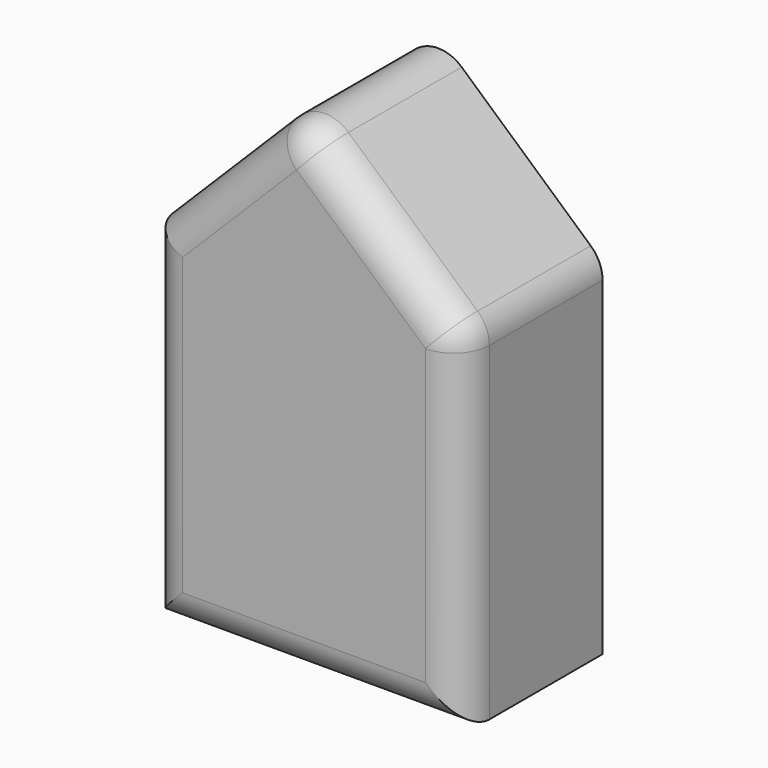
from build123d import *

# Parameters (mm, degrees)
F0_W     = 45.0788065791
F0_H     = 49.5671723038
F1_DEPTH = 25.4
F3_R     = 5.08


# Not quite as in the source:
# - a feature of the source that left no trace in its solid (it failed there, or was rolled back) is left out


with BuildPart() as f1:
    # F0 (on Front) → F1 (new body)
    with BuildSketch(Plane.XZ):
        with Locations((-4.0004998446, -2.9271943495)):
            Rectangle(F0_W, F0_H)
        Polygon((-5.2689509466, 43.1273430586), (-26.5399031341, 21.8563918024), (18.538903445, 21.8563918024), align=None)
    extrude(amount=F1_DEPTH)

    # F3
    f3_edges = [f1.edges().sort_by_distance(p)[0] for p in [
        (-15.904427, -25.4, 32.491867),
        (-26.539903, -25.4, -2.927194),
        (-4.0005, -25.4, -27.710781),
        (18.538903, -25.4, -2.927194),
        (6.634976, -25.4, 32.491867),
        (18.538903, -12.7, 21.856392),
        (-5.268951, -12.7, 43.127343),
    ]]
    fillet(f3_edges, radius=F3_R)


solid = f1.part
